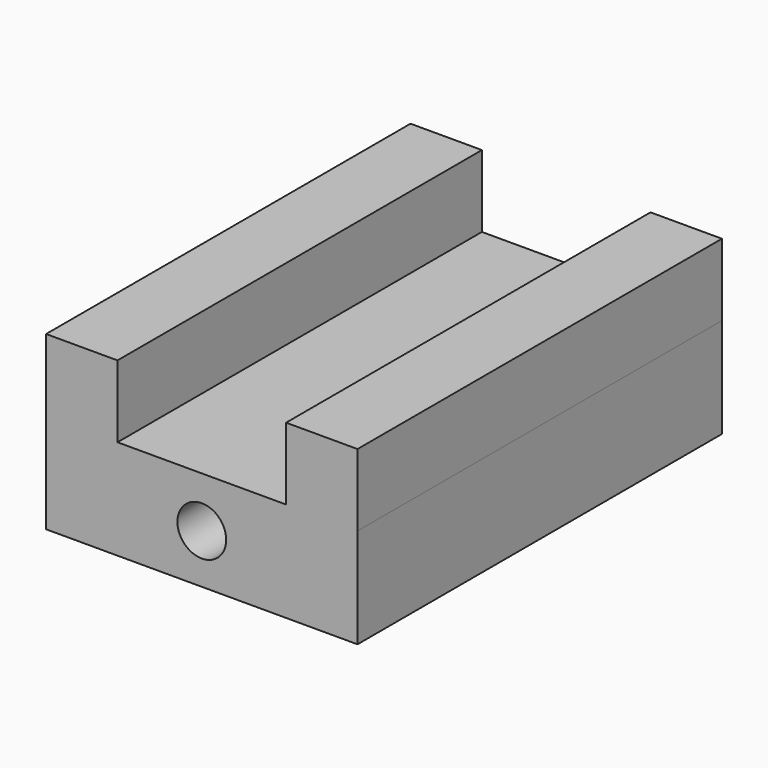
from build123d import *

# Parameters (mm, degrees)
F0_W     = 19.9103225023
F0_H     = 20.0946768746
F0_R     = 6.7973918103
F1_DEPTH = 63.5


# Not quite as in the source:
# - ends of sketch curves that miss each other by under 0.0002 mm in the source are joined


with BuildPart() as f1:
    # F0 (on Front) → F1 (new body, symmetric)
    with BuildSketch(Plane.XZ):
        with Locations((-33.4604037926, 24.1504837759)):
            Rectangle(F0_W, F0_H)
        Polygon((-23.5052425414, 14.1031453386), (-43.4155650437, 14.1031453386), (-43.4155650437, -13.7344365939), (43.4155575931, -13.7344365939), (43.4155575931, 14.1031453386), (23.5052425414, 14.1031453386), align=None)
        Circle(F0_R, mode=Mode.SUBTRACT)
        Polygon((23.5052425414, 34.1978222132), (23.5052425414, 14.1031453386), (43.4155575931, 14.1031453386), (43.4155650437, 34.1978222132), align=None)
    extrude(amount=F1_DEPTH, both=True)


solid = f1.part
